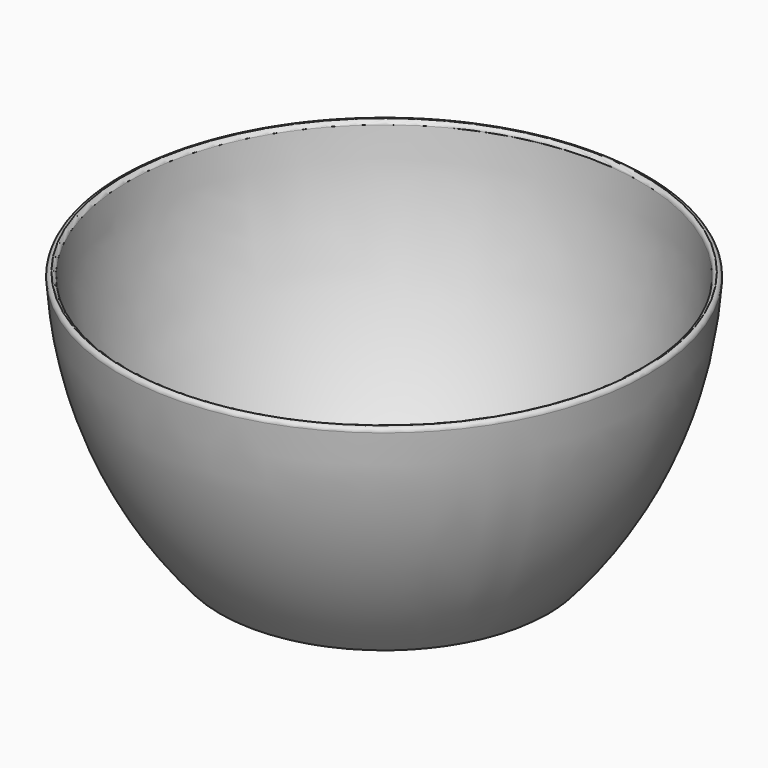
from build123d import *

# Parameters (mm, degrees)
F2_R = 0.1984375
F4_R = 0.1984375


# Not quite as in the source:
# - a fillet or chamfer that OpenCascade refuses, or shapes differently, is made with other operations: its cross-section is extruded or revolved along the edge and cut away or added


with BuildPart() as f1:
    # F0 (on Front) → F1 (revolve)
    with BuildSketch(Plane.XZ):
        with BuildLine():
            Line((7.7151542774, -11.6706086199), (0, -11.6706086199))
            Line((0, -11.6706086199), (0, -11.9529411765))
            Line((0, -11.9529411765), (7.8441176471, -11.9529411765))
            ThreePointArc((7.8441176471, -11.9529411765), (11.2904230804, -6.3901810676), (12.7, 0))
            Line((12.7, 0), (12.3264705882, 0))
            ThreePointArc((12.3264705882, 0), (11.0006527428, -6.2224609485), (7.7151542774, -11.6706086199))
        make_face()
    revolve(axis=Axis((0, 0, -5.9764705882), (0, 0, -1)))

    # F2
    f2_edges = [f1.edges().sort_by_distance(p)[0] for p in [
        (-12.7, 0, 0),
    ]]
    fillet(f2_edges, radius=F2_R)

    # F3: fillet of radius 0.1984375 on 1 edges, made by hand

    # F3_s1 → F3_t2 (revolve, cut)
    with BuildSketch(Plane.XZ):
        with BuildLine():
            ThreePointArc((12.490604679, 0), (12.3702545725, -0.0617556355), (12.3174431547, -0.1862902123))
            ThreePointArc((12.3174431547, -0.1862902123), (12.3221829622, -0.0931560623), (12.3264705882, 0))
            Line((12.3264705882, 0), (12.490604679, 0))
        make_face()
    revolve(axis=Axis((0, 0, 0), (0, 0, -1)), mode=Mode.SUBTRACT)

    # F4
    f4_edges = [f1.edges().sort_by_distance(p)[0] for p in [
        (-7.844118, 0, -11.952941),
    ]]
    fillet(f4_edges, radius=F4_R)


solid = f1.part
